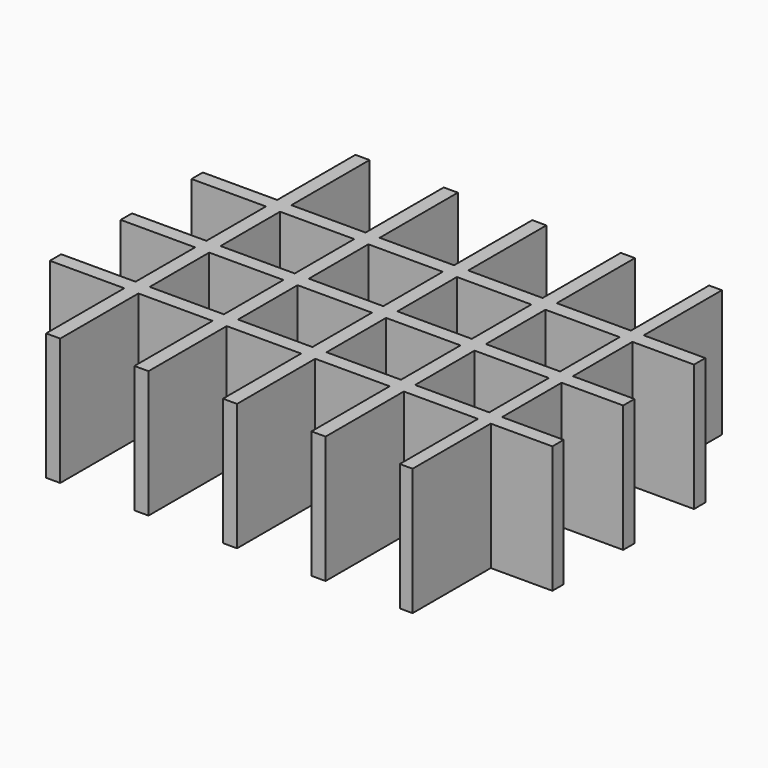
from build123d import *

# Parameters (mm, degrees)
F0_W     = 1.5
F0_H     = 10.375
F0_H_2   = 1.5
F0_W_2   = 7.9
F0_H_3   = 7.9
F0_W_3   = 7.875
F0_W_4   = 1.360903731
F0_W_5   = 6.539096269
F1_DEPTH = 13.5


with BuildPart() as f1:
    # F0 (on Top) → F1 (new body)
    with BuildSketch(Plane.XY):
        with Locations((-18.025, 15.3375)):
            Rectangle(F0_W, F0_H)
        with Locations((-18.025, 9.4)):
            Rectangle(F0_W, F0_H_2)
        with Locations((-22.725, 9.4)):
            Rectangle(F0_W_2, F0_H_2)
        with Locations((-18.025, 4.7)):
            Rectangle(F0_W, F0_H_3)
        with Locations((-18.025, 0)):
            Rectangle(F0_W, F0_H_2)
        with Locations((-22.725, 0)):
            Rectangle(F0_W_2, F0_H_2)
        with Locations((-18.025, -4.7)):
            Rectangle(F0_W, F0_H_3)
        with Locations((-18.025, -9.4)):
            Rectangle(F0_W, F0_H_2)
        with Locations((-22.725, -9.4)):
            Rectangle(F0_W_2, F0_H_2)
        with Locations((-18.025, -15.3375)):
            Rectangle(F0_W, F0_H)
        with Locations((-13.3375, -9.4)):
            Rectangle(F0_W_3, F0_H_2)
        with Locations((-8.65, -9.4)):
            Rectangle(F0_W, F0_H_2)
        with Locations((-8.65, -4.7)):
            Rectangle(F0_W, F0_H_3)
        with Locations((-8.65, 0)):
            Rectangle(F0_W, F0_H_2)
        with Locations((-13.3375, 0)):
            Rectangle(F0_W_3, F0_H_2)
        with Locations((-8.65, -15.3375)):
            Rectangle(F0_W, F0_H)
        with Locations((-8.65, 15.3375)):
            Rectangle(F0_W, F0_H)
        with Locations((-8.65, 9.4)):
            Rectangle(F0_W, F0_H_2)
        with Locations((-8.65, 4.7)):
            Rectangle(F0_W, F0_H_3)
        with Locations((-13.3375, 9.4)):
            Rectangle(F0_W_3, F0_H_2)
        with Locations((-3.95, 9.4)):
            Rectangle(F0_W_2, F0_H_2)
        with Locations((0.75, 9.4)):
            Rectangle(F0_W, F0_H_2)
        with Locations((0.75, 15.3375)):
            Rectangle(F0_W, F0_H)
        with Locations((0.75, 4.7)):
            Rectangle(F0_W, F0_H_3)
        with Locations((-3.95, 0)):
            Rectangle(F0_W_2, F0_H_2)
        with Locations((0.75, 0)):
            Rectangle(F0_W, F0_H_2)
        with Locations((0.75, -4.7)):
            Rectangle(F0_W, F0_H_3)
        with Locations((0.75, -9.4)):
            Rectangle(F0_W, F0_H_2)
        with Locations((-3.95, -9.4)):
            Rectangle(F0_W_2, F0_H_2)
        with Locations((0.75, -15.3375)):
            Rectangle(F0_W, F0_H)
        with Locations((5.45, -9.4)):
            Rectangle(F0_W_2, F0_H_2)
        with Locations((10.15, -15.3375)):
            Rectangle(F0_W, F0_H)
        with Locations((19.4554518655, -15.3375)):
            Rectangle(F0_W_4, F0_H)
        with Locations((23.4054518655, -9.4)):
            Rectangle(F0_W_5, F0_H_2)
        with Locations((14.8375, -9.4)):
            Rectangle(F0_W_3, F0_H_2)
        with Locations((19.4554518655, -9.4)):
            Rectangle(F0_W_4, F0_H_2)
        with Locations((10.15, -9.4)):
            Rectangle(F0_W, F0_H_2)
        with Locations((10.15, -4.7)):
            Rectangle(F0_W, F0_H_3)
        with Locations((19.4554518655, -4.7)):
            Rectangle(F0_W_4, F0_H_3)
        with Locations((19.4554518655, 0)):
            Rectangle(F0_W_4, F0_H_2)
        with Locations((14.8375, 0)):
            Rectangle(F0_W_3, F0_H_2)
        with Locations((10.15, 0)):
            Rectangle(F0_W, F0_H_2)
        with Locations((5.45, 0)):
            Rectangle(F0_W_2, F0_H_2)
        with Locations((19.4554518655, 4.7)):
            Rectangle(F0_W_4, F0_H_3)
        with Locations((10.15, 4.7)):
            Rectangle(F0_W, F0_H_3)
        with Locations((23.4054518655, 0)):
            Rectangle(F0_W_5, F0_H_2)
        with Locations((23.4054518655, 9.4)):
            Rectangle(F0_W_5, F0_H_2)
        with Locations((14.8375, 9.4)):
            Rectangle(F0_W_3, F0_H_2)
        with Locations((19.4554518655, 9.4)):
            Rectangle(F0_W_4, F0_H_2)
        with Locations((19.4554518655, 15.3375)):
            Rectangle(F0_W_4, F0_H)
        with Locations((10.15, 15.3375)):
            Rectangle(F0_W, F0_H)
        with Locations((10.15, 9.4)):
            Rectangle(F0_W, F0_H_2)
        with Locations((5.45, 9.4)):
            Rectangle(F0_W_2, F0_H_2)
    extrude(amount=F1_DEPTH)


solid = f1.part
